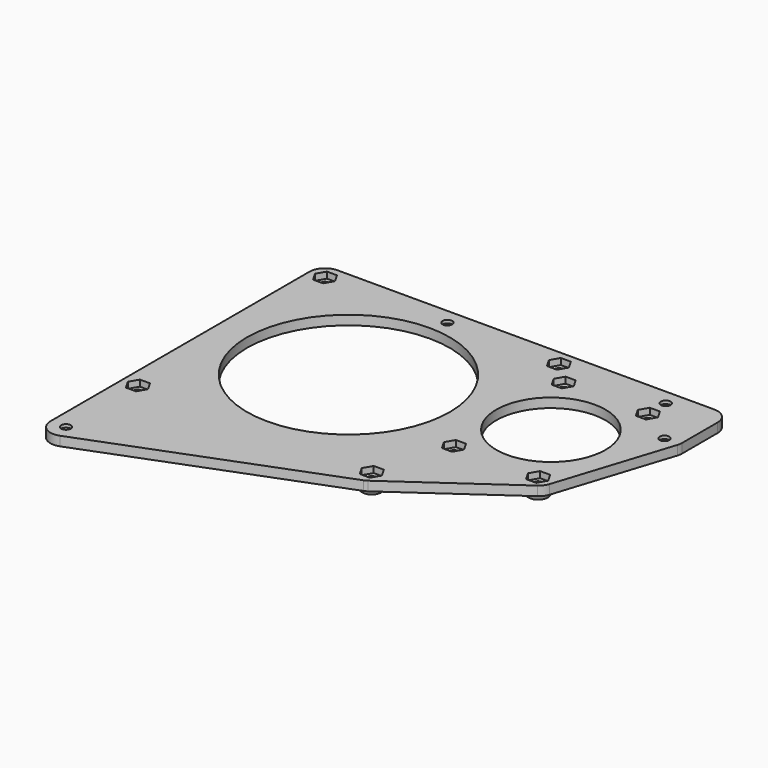
from build123d import *

# Parameters (mm, degrees)
F0_R      = 1.55
F0_R_2    = 32.5
F0_R_3    = 17.5
F1_DEPTH  = 3
F2_R      = 3.5
F3_DEPTH  = 2
F4_R      = 0.99999
F6_DEPTH  = 2
F7_R      = 1.55
F8_DEPTH  = 25
F10_DEPTH = 2


# Not quite as in the source:
# - a fillet or chamfer is up to 0.001 mm smaller than in the source, because OpenCascade refuses the exact size


with BuildPart() as f1:
    # F0 (on Top) → F1 (new body)
    with BuildSketch(Plane.XY):
        with BuildLine():
            Line((57.9264685896, 61.5924972273), (-62.9658055305, 61.5924972273))
            ThreePointArc((-62.9658055305, 61.5924972273), (-66.5013394365, 60.1280311332), (-67.9658055305, 56.5924972273))
            Line((-67.9658055305, 56.5924972273), (-67.9658055305, -47.2312074405))
            ThreePointArc((-67.9658055305, -47.2312074405), (-65.7970250714, -51.3523960933), (-61.1721271659, -51.8984033786))
            Line((-61.1721271659, -51.8984033786), (13.2519902581, -23.2960196347))
            ThreePointArc((13.2519902581, -23.2960196347), (13.8100380076, -23.0412362209), (14.332684577, -22.7200315472))
            Line((14.332684577, -22.7200315472), (49.0800604394, 1.6925408888))
            ThreePointArc((49.0800604394, 1.6925408888), (50.2332004004, 2.8207870625), (50.967048715, 4.2574978369))
            Line((50.967048715, 4.2574978369), (62.6878295487, 40.8221728745))
            ThreePointArc((62.6878295487, 40.8221728745), (62.8664485894, 41.5760264684), (62.9264685896, 42.3484237769))
            Line((62.9264685896, 42.3484237769), (62.9264685896, 56.5924972273))
            ThreePointArc((62.9264685896, 56.5924972273), (61.4620024956, 60.1280311332), (57.9264685896, 61.5924972273))
        make_face()
        with Locations((-62.9658055305, -47.2312074405)):
            Circle(F0_R, mode=Mode.SUBTRACT)
        with Locations((-25.4658055305, 19.0924972273)):
            Circle(F0_R_2, mode=Mode.SUBTRACT)
        with Locations((-23.702102839, 56.5924972273)):
            Circle(F0_R, mode=Mode.SUBTRACT)
        with Locations((32.797897161, 27.4372637533)):
            Circle(F0_R_3, mode=Mode.SUBTRACT)
        with Locations((57.9264685896, 41.5666419594)):
            Circle(F0_R, mode=Mode.SUBTRACT)
        with Locations((46.297897161, 56.5924972273)):
            Circle(F0_R, mode=Mode.SUBTRACT)
    extrude(amount=F1_DEPTH)

    # F2 (on face) → F3 (join)
    with BuildSketch(Plane(origin=(0, 0, 0), x_dir=(1, 0, 0), z_dir=(0, 0, -1))):
        with Locations((-62.9658055305, -56.5924972273)):
            Circle(F2_R)
        with Locations((12.0341944695, -56.5924972273)):
            Circle(F2_R)
        with Locations((12.0341944695, 18.4075027727)):
            Circle(F2_R)
        with Locations((-62.9658055305, 18.4075027727)):
            Circle(F2_R)
        with Locations((19.297897161, -49.4372637533)):
            Circle(F2_R)
        with Locations((46.297897161, -49.4372637533)):
            Circle(F2_R)
        with Locations((46.297897161, -5.4372637533)):
            Circle(F2_R)
        with Locations((19.297897161, -5.4372637533)):
            Circle(F2_R)
    extrude(amount=F3_DEPTH)

    # F4 (radius 1 in the source; OpenCascade refuses exactly that, so slightly less here)
    f4_edges = [f1.edges().sort_by_distance(p)[0] for p in [
        (-59.465806, -18.407503, -1),
        (-66.465806, -18.407503, 0),
        (-66.465806, -18.407503, -2),
        (-59.465806, 56.592497, -1),
        (-66.465806, 56.592497, 0),
        (-66.465806, 56.592497, -2),
        (15.534194, -18.407503, -1),
        (8.534194, -18.407503, 0),
        (8.534194, -18.407503, -2),
        (22.797897, 5.437264, -1),
        (15.797897, 5.437264, 0),
        (15.797897, 5.437264, -2),
        (22.797897, 49.437264, -1),
        (15.797897, 49.437264, 0),
        (15.797897, 49.437264, -2),
        (15.534194, 56.592497, -1),
        (8.534194, 56.592497, 0),
        (8.534194, 56.592497, -2),
        (49.797897, 5.437264, -1),
        (42.797897, 5.437264, 0),
        (42.797897, 5.437264, -2),
        (49.797897, 49.437264, -1),
        (42.797897, 49.437264, 0),
        (42.797897, 49.437264, -2),
    ]]
    fillet(f4_edges, radius=F4_R)

    # F5 (on face) → F6 (cut)
    with BuildSketch(Plane.XY.offset(3)):
        Polygon((-64.5823862843, -21.2075027727), (-61.3492247768, -21.2075027727), (-59.7326440231, -18.4075027727), (-61.3492247768, -15.6075027727), (-64.5823862843, -15.6075027727), (-66.198967038, -18.4075027727), align=None)
        Polygon((10.4176137157, -21.2075027727), (13.6507752232, -21.2075027727), (15.2673559769, -18.4075027727), (13.6507752232, -15.6075027727), (10.4176137157, -15.6075027727), (8.801032962, -18.4075027727), align=None)
        Polygon((17.6813164073, 2.6372637533), (20.9144779148, 2.6372637533), (22.5310586685, 5.4372637533), (20.9144779148, 8.2372637533), (17.6813164073, 8.2372637533), (16.0647356536, 5.4372637533), align=None)
        Polygon((-64.5823862843, 53.7924972273), (-61.3492247768, 53.7924972273), (-59.7326440231, 56.5924972273), (-61.3492247768, 59.3924972273), (-64.5823862843, 59.3924972273), (-66.198967038, 56.5924972273), align=None)
        Polygon((10.4176137157, 53.7924972273), (13.6507752232, 53.7924972273), (15.2673559769, 56.5924972273), (13.6507752232, 59.3924972273), (10.4176137157, 59.3924972273), (8.801032962, 56.5924972273), align=None)
        Polygon((17.6813164073, 46.6372637533), (20.9144779148, 46.6372637533), (22.5310586685, 49.4372637533), (20.9144779148, 52.2372637533), (17.6813164073, 52.2372637533), (16.0647356536, 49.4372637533), align=None)
        Polygon((44.6813164073, 46.6372637533), (47.9144779148, 46.6372637533), (49.5310586685, 49.4372637533), (47.9144779148, 52.2372637533), (44.6813164073, 52.2372637533), (43.0647356536, 49.4372637533), align=None)
        Polygon((47.9144779148, 8.2372637533), (44.6813164073, 8.2372637533), (43.0647356536, 5.4372637533), (44.6813164073, 2.6372637533), (47.9144779148, 2.6372637533), (49.5310586685, 5.4372637533), align=None)
    extrude(amount=-F6_DEPTH, mode=Mode.SUBTRACT)

    # F7 (on face) → F8 (cut)
    with BuildSketch(Plane.XY.offset(3)):
        with Locations((-62.9658055305, 56.5924972273)):
            Circle(F7_R)
        with Locations((-62.9658055305, -18.4075027727)):
            Circle(F7_R)
        with Locations((19.297897161, 5.4372637533)):
            Circle(F7_R)
        with Locations((46.297897161, 5.4372637533)):
            Circle(F7_R)
        with Locations((46.297897161, 49.4372637533)):
            Circle(F7_R)
        with Locations((19.297897161, 49.4372637533)):
            Circle(F7_R)
        with Locations((12.0341944695, -18.4075027727)):
            Circle(F7_R)
        with Locations((12.0341944695, 56.5924972273)):
            Circle(F7_R)
    extrude(amount=-F8_DEPTH, mode=Mode.SUBTRACT)

    # F9 (on face) → F10 (cut)
    with BuildSketch(Plane(origin=(0, 0, 0), x_dir=(1, 0, 0), z_dir=(0, 0, -1))):
        Polygon((-64.5823862843, 44.4312074405), (-61.3492247768, 44.4312074405), (-59.7326440231, 47.2312074405), (-61.3492247768, 50.0312074405), (-64.5823862843, 50.0312074405), (-66.198967038, 47.2312074405), align=None)
        Polygon((-25.3186835927, -59.3924972273), (-22.0855220852, -59.3924972273), (-20.4689413315, -56.5924972273), (-22.0855220852, -53.7924972273), (-25.3186835927, -53.7924972273), (-26.9352643464, -56.5924972273), align=None)
        Polygon((44.6813164073, -59.3924972273), (47.9144779148, -59.3924972273), (49.5310586685, -56.5924972273), (47.9144779148, -53.7924972273), (44.6813164073, -53.7924972273), (43.0647356536, -56.5924972273), align=None)
        Polygon((56.3098878359, -44.3666419594), (59.5430493434, -44.3666419594), (61.1596300971, -41.5666419594), (59.5430493434, -38.7666419594), (56.3098878359, -38.7666419594), (54.6933070822, -41.5666419594), align=None)
    extrude(amount=-F10_DEPTH, mode=Mode.SUBTRACT)


solid = f1.part
